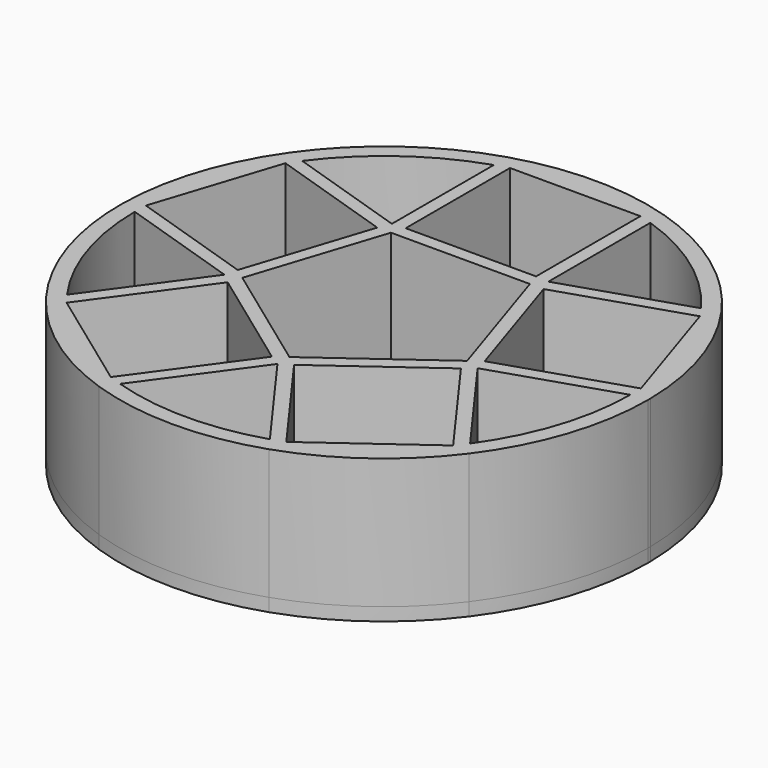
from build123d import *
from build123d import SkipClean  # not in build123d's __all__

# Parameters (mm, degrees)
F0_W     = 10
F0_H     = 10
F1_DEPTH = 1
F2_DEPTH = 10


with BuildPart() as f1:
    # F0 (on Top) → F1 (new body)
    with BuildSketch(Plane.XY):
        with BuildLine():
            Line((6, 8.2582915228), (6, 18.0277563773))
            ThreePointArc((6, 18.0277563773), (5.5020799323, 18.1859043333), (5, 18.3303027798))
            Line((5, 18.3303027798), (5, 8.3303027798))
            Line((5, 8.3303027798), (-5, 8.3303027798))
            Line((-5, 8.3303027798), (-5, 18.3303027798))
            ThreePointArc((-5, 18.3303027798), (-5.5020799323, 18.1859043333), (-6, 18.0277563773))
            Line((-6, 18.0277563773), (-6, 8.2582915228))
            Line((-6, 8.2582915228), (-5.1174302589, 7.9715272307))
            Line((-5.1174302589, 7.9715272307), (-5.3257767127, 7.3303027798))
            Line((-5.3257767127, 7.3303027798), (5.3257767127, 7.3303027798))
            Line((5.3257767127, 7.3303027798), (5.1174302589, 7.9715272307))
            Line((5.1174302589, 7.9715272307), (6, 8.2582915228))
        make_face()
        with BuildLine():
            ThreePointArc((-6.5079649301, -19.165254969), (0, -20.2400742479), (6.5079649301, -19.165254969))
            Line((6.5079649301, -19.165254969), (5.7423473643, -18.1114727935))
            ThreePointArc((5.7423473643, -18.1114727935), (0, -19), (-5.7423473643, -18.1114727935))
            Line((-5.7423473643, -18.1114727935), (-6.5079649301, -19.165254969))
        make_face()
        with BuildLine():
            ThreePointArc((-6.7291966722, -17.7684527224), (-6.2381301971, -17.9467471048), (-5.7423473643, -18.1114727935))
            Line((-5.7423473643, -18.1114727935), (0, -10.2078097002))
            Line((0, -10.2078097002), (-0.5454580974, -9.4570510365))
            Line((-0.5454580974, -9.4570510365), (0, -9.0607525315))
            Line((0, -9.0607525315), (-8.6172877376, -2.7999265141))
            Line((-8.6172877376, -2.7999265141), (-8.8256341914, -3.4411509649))
            Line((-8.8256341914, -3.4411509649), (-9.7082039325, -3.1543866727))
            Line((-9.7082039325, -3.1543866727), (-15.4505512968, -11.0580497659))
            ThreePointArc((-15.4505512968, -11.0580497659), (-15.1406825363, -11.4786642225), (-14.8193666159, -11.8906001995))
            Line((-14.8193666159, -11.8906001995), (-8.941514093, -3.8004302557))
            Line((-8.941514093, -3.8004302557), (-0.8513441492, -9.6782827786))
            Line((-0.8513441492, -9.6782827786), (-6.7291966722, -17.7684527224))
        make_face()
        Polygon((18.9782388763, 0.9090924895), (15.8880689325, 10.4196576525), (6.3775037696, 7.3294877087), (9.4676737133, -2.1810774542), align=None)
        Polygon((0, -9.0607525315), (8.6172877376, -2.7999265141), (5.3257767127, 7.3303027798), (-5.3257767127, 7.3303027798), (-8.6172877376, -2.7999265141), align=None)
        with BuildLine():
            Line((6, 8.2582915228), (15.2913132106, 11.2772221888))
            ThreePointArc((15.2913132106, 11.2772221888), (11.1679197936, 15.3713228931), (6, 18.0277563773))
            Line((6, 18.0277563773), (6, 8.2582915228))
        make_face()
        Polygon((-6.3775037696, 7.3294877087), (-15.8880689325, 10.4196576525), (-18.9782388763, 0.9090924895), (-9.4676737133, -2.1810774542), align=None)
        with BuildLine():
            ThreePointArc((16.2161688626, -12.1118319415), (19.2077727412, -6.3813847935), (20.2400742479, 0))
            ThreePointArc((20.2400742479, 0), (20.2396337779, 0.1335293897), (20.238312387, 0.2670529676))
            Line((20.238312387, 0.2670529676), (18.9995171431, -0.1354560067))
            ThreePointArc((18.9995171431, -0.1354560067), (18.0700738096, -5.8713228931), (15.4505512968, -11.0580497659))
            Line((15.4505512968, -11.0580497659), (16.2161688626, -12.1118319415))
        make_face()
        with BuildLine():
            ThreePointArc((14.8193666159, -11.8906001995), (15.1406825363, -11.4786642225), (15.4505512968, -11.0580497659))
            Line((15.4505512968, -11.0580497659), (9.7082039325, -3.1543866727))
            Line((9.7082039325, -3.1543866727), (8.8256341914, -3.4411509649))
            Line((8.8256341914, -3.4411509649), (8.6172877376, -2.7999265141))
            Line((8.6172877376, -2.7999265141), (0, -9.0607525315))
            Line((0, -9.0607525315), (0.5454580974, -9.4570510365))
            Line((0.5454580974, -9.4570510365), (0, -10.2078097002))
            Line((0, -10.2078097002), (5.7423473643, -18.1114727935))
            ThreePointArc((5.7423473643, -18.1114727935), (6.2381301971, -17.9467471048), (6.7291966722, -17.7684527224))
            Line((6.7291966722, -17.7684527224), (0.8513441492, -9.6782827786))
            Line((0.8513441492, -9.6782827786), (8.941514093, -3.8004302557))
            Line((8.941514093, -3.8004302557), (14.8193666159, -11.8906001995))
        make_face()
        with BuildLine():
            Line((-6, 18.0277563773), (-6, 19.3303027798))
            ThreePointArc((-6, 19.3303027798), (-11.8968171482, 16.3745640339), (-16.5301084545, 11.6797311631))
            Line((-16.5301084545, 11.6797311631), (-15.2913132106, 11.2772221888))
            ThreePointArc((-15.2913132106, 11.2772221888), (-11.1679197936, 15.3713228931), (-6, 18.0277563773))
        make_face()
        with BuildLine():
            ThreePointArc((-18.9995171431, -0.1354560067), (-18.0700738096, -5.8713228931), (-15.4505512968, -11.0580497659))
            Line((-15.4505512968, -11.0580497659), (-9.7082039325, -3.1543866727))
            Line((-9.7082039325, -3.1543866727), (-18.9995171431, -0.1354560067))
        make_face()
        with Locations((0, 13.3303027798)):
            Rectangle(F0_W, F0_H)
        with BuildLine():
            ThreePointArc((6.5079649301, -19.165254969), (11.8968171482, -16.3745640339), (16.2161688626, -12.1118319415))
            Line((16.2161688626, -12.1118319415), (6.5079649301, -19.165254969))
        make_face()
        with BuildLine():
            ThreePointArc((-16.2161688626, -12.1118319415), (-11.8968171482, -16.3745640339), (-6.5079649301, -19.165254969))
            Line((-6.5079649301, -19.165254969), (-16.2161688626, -12.1118319415))
        make_face()
        with BuildLine():
            Line((-20.238312387, 0.2670529676), (-16.5301084545, 11.6797311631))
            ThreePointArc((-16.5301084545, 11.6797311631), (-19.2494545037, 6.25452691), (-20.238312387, 0.2670529676))
        make_face()
        with BuildLine():
            Line((-6, 19.3303027798), (6, 19.3303027798))
            ThreePointArc((6, 19.3303027798), (0, 20.2400742479), (-6, 19.3303027798))
        make_face()
        with BuildLine():
            Line((16.5301084545, 11.6797311631), (20.238312387, 0.2670529676))
            ThreePointArc((20.238312387, 0.2670529676), (19.2494545037, 6.25452691), (16.5301084545, 11.6797311631))
        make_face()
        with BuildLine():
            Line((-15.2913132106, 11.2772221888), (-16.5301084545, 11.6797311631))
            Line((-16.5301084545, 11.6797311631), (-20.238312387, 0.2670529676))
            Line((-20.238312387, 0.2670529676), (-18.9995171431, -0.1354560067))
            ThreePointArc((-18.9995171431, -0.1354560067), (-18.9960590244, 0.3869645243), (-18.9782388763, 0.9090924895))
            ThreePointArc((-18.9782388763, 0.9090924895), (-18.0700738096, 5.8713228931), (-15.8880689325, 10.4196576525))
            ThreePointArc((-15.8880689325, 10.4196576525), (-15.5955866174, 10.8525424698), (-15.2913132106, 11.2772221888))
        make_face()
        Polygon((-14.8193666159, -11.8906001995), (-6.7291966722, -17.7684527224), (-0.8513441492, -9.6782827786), (-8.941514093, -3.8004302557), align=None)
        with BuildLine():
            Line((9.7082039325, -3.1543866727), (18.9995171431, -0.1354560067))
            ThreePointArc((18.9995171431, -0.1354560067), (18.9998792854, -0.0677284337), (19, 0))
            ThreePointArc((19, 0), (18.99455894, 0.4546764512), (18.9782388763, 0.9090924895))
            Line((18.9782388763, 0.9090924895), (9.4676737133, -2.1810774542))
            Line((9.4676737133, -2.1810774542), (6.3775037696, 7.3294877087))
            Line((6.3775037696, 7.3294877087), (15.8880689325, 10.4196576525))
            ThreePointArc((15.8880689325, 10.4196576525), (15.5955866174, 10.8525424698), (15.2913132106, 11.2772221888))
            Line((15.2913132106, 11.2772221888), (6, 8.2582915228))
            Line((6, 8.2582915228), (6, 7.3303027798))
            Line((6, 7.3303027798), (5.3257767127, 7.3303027798))
            Line((5.3257767127, 7.3303027798), (8.6172877376, -2.7999265141))
            Line((8.6172877376, -2.7999265141), (9.1627458351, -2.403628009))
            Line((9.1627458351, -2.403628009), (9.7082039325, -3.1543866727))
        make_face()
        with BuildLine():
            ThreePointArc((15.4505512968, -11.0580497659), (18.0700738096, -5.8713228931), (18.9995171431, -0.1354560067))
            Line((18.9995171431, -0.1354560067), (9.7082039325, -3.1543866727))
            Line((9.7082039325, -3.1543866727), (15.4505512968, -11.0580497659))
        make_face()
        with BuildLine():
            ThreePointArc((-20.238312387, 0.2670529676), (-19.2494545037, -6.25452691), (-16.2161688626, -12.1118319415))
            Line((-16.2161688626, -12.1118319415), (-15.4505512968, -11.0580497659))
            ThreePointArc((-15.4505512968, -11.0580497659), (-18.0700738096, -5.8713228931), (-18.9995171431, -0.1354560067))
            Line((-18.9995171431, -0.1354560067), (-20.238312387, 0.2670529676))
        make_face()
        with BuildLine():
            Line((-6, 8.2582915228), (-15.2913132106, 11.2772221888))
            ThreePointArc((-15.2913132106, 11.2772221888), (-15.5955866174, 10.8525424698), (-15.8880689325, 10.4196576525))
            Line((-15.8880689325, 10.4196576525), (-6.3775037696, 7.3294877087))
            Line((-6.3775037696, 7.3294877087), (-9.4676737133, -2.1810774542))
            Line((-9.4676737133, -2.1810774542), (-18.9782388763, 0.9090924895))
            ThreePointArc((-18.9782388763, 0.9090924895), (-18.9960590244, 0.3869645243), (-18.9995171431, -0.1354560067))
            Line((-18.9995171431, -0.1354560067), (-9.7082039325, -3.1543866727))
            Line((-9.7082039325, -3.1543866727), (-9.1627458351, -2.403628009))
            Line((-9.1627458351, -2.403628009), (-8.6172877376, -2.7999265141))
            Line((-8.6172877376, -2.7999265141), (-5.3257767127, 7.3303027798))
            Line((-5.3257767127, 7.3303027798), (-6, 7.3303027798))
            Line((-6, 7.3303027798), (-6, 8.2582915228))
        make_face()
        with BuildLine():
            Line((15.2913132106, 11.2772221888), (16.5301084545, 11.6797311631))
            ThreePointArc((16.5301084545, 11.6797311631), (11.8968171482, 16.3745640339), (6, 19.3303027798))
            Line((6, 19.3303027798), (6, 18.0277563773))
            ThreePointArc((6, 18.0277563773), (11.1679197936, 15.3713228931), (15.2913132106, 11.2772221888))
        make_face()
        Polygon((6.7291966722, -17.7684527224), (14.8193666159, -11.8906001995), (8.941514093, -3.8004302557), (0.8513441492, -9.6782827786), align=None)
        with BuildLine():
            ThreePointArc((-5.7423473643, -18.1114727935), (0, -19), (5.7423473643, -18.1114727935))
            Line((5.7423473643, -18.1114727935), (0, -10.2078097002))
            Line((0, -10.2078097002), (-5.7423473643, -18.1114727935))
        make_face()
        with BuildLine():
            Line((-6, 8.2582915228), (-6, 18.0277563773))
            ThreePointArc((-6, 18.0277563773), (-11.1679197936, 15.3713228931), (-15.2913132106, 11.2772221888))
            Line((-15.2913132106, 11.2772221888), (-6, 8.2582915228))
        make_face()
        with BuildLine():
            Line((18.9995171431, -0.1354560067), (20.238312387, 0.2670529676))
            Line((20.238312387, 0.2670529676), (16.5301084545, 11.6797311631))
            Line((16.5301084545, 11.6797311631), (15.2913132106, 11.2772221888))
            ThreePointArc((15.2913132106, 11.2772221888), (15.5955866174, 10.8525424698), (15.8880689325, 10.4196576525))
            ThreePointArc((15.8880689325, 10.4196576525), (18.0700738096, 5.8713228931), (18.9782388763, 0.9090924895))
            ThreePointArc((18.9782388763, 0.9090924895), (18.99455894, 0.4546764512), (19, 0))
            ThreePointArc((19, 0), (18.9998792854, -0.0677284337), (18.9995171431, -0.1354560067))
        make_face()
        with BuildLine():
            Line((6, 18.0277563773), (6, 19.3303027798))
            Line((6, 19.3303027798), (-6, 19.3303027798))
            Line((-6, 19.3303027798), (-6, 18.0277563773))
            ThreePointArc((-6, 18.0277563773), (-5.5020799323, 18.1859043333), (-5, 18.3303027798))
            ThreePointArc((-5, 18.3303027798), (0, 19), (5, 18.3303027798))
            ThreePointArc((5, 18.3303027798), (5.5020799323, 18.1859043333), (6, 18.0277563773))
        make_face()
        with BuildLine():
            Line((6.5079649301, -19.165254969), (16.2161688626, -12.1118319415))
            Line((16.2161688626, -12.1118319415), (15.4505512968, -11.0580497659))
            ThreePointArc((15.4505512968, -11.0580497659), (15.1406825363, -11.4786642225), (14.8193666159, -11.8906001995))
            ThreePointArc((14.8193666159, -11.8906001995), (11.1679197936, -15.3713228931), (6.7291966722, -17.7684527224))
            ThreePointArc((6.7291966722, -17.7684527224), (6.2381301971, -17.9467471048), (5.7423473643, -18.1114727935))
            Line((5.7423473643, -18.1114727935), (6.5079649301, -19.165254969))
        make_face()
        with BuildLine():
            Line((-16.2161688626, -12.1118319415), (-6.5079649301, -19.165254969))
            Line((-6.5079649301, -19.165254969), (-5.7423473643, -18.1114727935))
            ThreePointArc((-5.7423473643, -18.1114727935), (-6.2381301971, -17.9467471048), (-6.7291966722, -17.7684527224))
            ThreePointArc((-6.7291966722, -17.7684527224), (-11.1679197936, -15.3713228931), (-14.8193666159, -11.8906001995))
            ThreePointArc((-14.8193666159, -11.8906001995), (-15.1406825363, -11.4786642225), (-15.4505512968, -11.0580497659))
            Line((-15.4505512968, -11.0580497659), (-16.2161688626, -12.1118319415))
        make_face()
        with BuildLine():
            ThreePointArc((6.7291966722, -17.7684527224), (11.1679197936, -15.3713228931), (14.8193666159, -11.8906001995))
            Line((14.8193666159, -11.8906001995), (6.7291966722, -17.7684527224))
        make_face()
        with BuildLine():
            ThreePointArc((-14.8193666159, -11.8906001995), (-11.1679197936, -15.3713228931), (-6.7291966722, -17.7684527224))
            Line((-6.7291966722, -17.7684527224), (-14.8193666159, -11.8906001995))
        make_face()
        with BuildLine():
            Line((-18.9782388763, 0.9090924895), (-15.8880689325, 10.4196576525))
            ThreePointArc((-15.8880689325, 10.4196576525), (-18.0700738096, 5.8713228931), (-18.9782388763, 0.9090924895))
        make_face()
        with BuildLine():
            Line((-5, 18.3303027798), (5, 18.3303027798))
            ThreePointArc((5, 18.3303027798), (0, 19), (-5, 18.3303027798))
        make_face()
        with BuildLine():
            ThreePointArc((18.9782388763, 0.9090924895), (18.0700738096, 5.8713228931), (15.8880689325, 10.4196576525))
            Line((15.8880689325, 10.4196576525), (18.9782388763, 0.9090924895))
        make_face()
        Polygon((8.8256341914, -3.4411509649), (9.7082039325, -3.1543866727), (9.1627458351, -2.403628009), (8.6172877376, -2.7999265141), align=None)
        Polygon((6, 7.3303027798), (6, 8.2582915228), (5.1174302589, 7.9715272307), (5.3257767127, 7.3303027798), align=None)
        Polygon((-5.1174302589, 7.9715272307), (-6, 8.2582915228), (-6, 7.3303027798), (-5.3257767127, 7.3303027798), align=None)
        Polygon((-9.1627458351, -2.403628009), (-9.7082039325, -3.1543866727), (-8.8256341914, -3.4411509649), (-8.6172877376, -2.7999265141), align=None)
        Polygon((-0.5454580974, -9.4570510365), (0, -10.2078097002), (0.5454580974, -9.4570510365), (0, -9.0607525315), align=None)
    extrude(amount=-F1_DEPTH)

    # F0 (on Top) → F2 (join)
    with BuildSketch(Plane.XY):
        with BuildLine():
            Line((-6, 18.0277563773), (-6, 19.3303027798))
            ThreePointArc((-6, 19.3303027798), (-11.8968171482, 16.3745640339), (-16.5301084545, 11.6797311631))
            Line((-16.5301084545, 11.6797311631), (-15.2913132106, 11.2772221888))
            ThreePointArc((-15.2913132106, 11.2772221888), (-11.1679197936, 15.3713228931), (-6, 18.0277563773))
        make_face()
        with BuildLine():
            Line((6, 8.2582915228), (6, 18.0277563773))
            ThreePointArc((6, 18.0277563773), (5.5020799323, 18.1859043333), (5, 18.3303027798))
            Line((5, 18.3303027798), (5, 8.3303027798))
            Line((5, 8.3303027798), (-5, 8.3303027798))
            Line((-5, 8.3303027798), (-5, 18.3303027798))
            ThreePointArc((-5, 18.3303027798), (-5.5020799323, 18.1859043333), (-6, 18.0277563773))
            Line((-6, 18.0277563773), (-6, 8.2582915228))
            Line((-6, 8.2582915228), (-5.1174302589, 7.9715272307))
            Line((-5.1174302589, 7.9715272307), (-5.3257767127, 7.3303027798))
            Line((-5.3257767127, 7.3303027798), (5.3257767127, 7.3303027798))
            Line((5.3257767127, 7.3303027798), (5.1174302589, 7.9715272307))
            Line((5.1174302589, 7.9715272307), (6, 8.2582915228))
        make_face()
        with BuildLine():
            Line((-18.9782388763, 0.9090924895), (-15.8880689325, 10.4196576525))
            ThreePointArc((-15.8880689325, 10.4196576525), (-18.0700738096, 5.8713228931), (-18.9782388763, 0.9090924895))
        make_face()
        with BuildLine():
            Line((-5, 18.3303027798), (5, 18.3303027798))
            ThreePointArc((5, 18.3303027798), (0, 19), (-5, 18.3303027798))
        make_face()
        with BuildLine():
            ThreePointArc((18.9782388763, 0.9090924895), (18.0700738096, 5.8713228931), (15.8880689325, 10.4196576525))
            Line((15.8880689325, 10.4196576525), (18.9782388763, 0.9090924895))
        make_face()
        with BuildLine():
            Line((-20.238312387, 0.2670529676), (-16.5301084545, 11.6797311631))
            ThreePointArc((-16.5301084545, 11.6797311631), (-19.2494545037, 6.25452691), (-20.238312387, 0.2670529676))
        make_face()
        with BuildLine():
            Line((-6, 19.3303027798), (6, 19.3303027798))
            ThreePointArc((6, 19.3303027798), (0, 20.2400742479), (-6, 19.3303027798))
        make_face()
        with BuildLine():
            Line((16.5301084545, 11.6797311631), (20.238312387, 0.2670529676))
            ThreePointArc((20.238312387, 0.2670529676), (19.2494545037, 6.25452691), (16.5301084545, 11.6797311631))
        make_face()
        with BuildLine():
            Line((-15.2913132106, 11.2772221888), (-16.5301084545, 11.6797311631))
            Line((-16.5301084545, 11.6797311631), (-20.238312387, 0.2670529676))
            Line((-20.238312387, 0.2670529676), (-18.9995171431, -0.1354560067))
            ThreePointArc((-18.9995171431, -0.1354560067), (-18.9960590244, 0.3869645243), (-18.9782388763, 0.9090924895))
            ThreePointArc((-18.9782388763, 0.9090924895), (-18.0700738096, 5.8713228931), (-15.8880689325, 10.4196576525))
            ThreePointArc((-15.8880689325, 10.4196576525), (-15.5955866174, 10.8525424698), (-15.2913132106, 11.2772221888))
        make_face()
        with BuildLine():
            Line((9.7082039325, -3.1543866727), (18.9995171431, -0.1354560067))
            ThreePointArc((18.9995171431, -0.1354560067), (18.9998792854, -0.0677284337), (19, 0))
            ThreePointArc((19, 0), (18.99455894, 0.4546764512), (18.9782388763, 0.9090924895))
            Line((18.9782388763, 0.9090924895), (9.4676737133, -2.1810774542))
            Line((9.4676737133, -2.1810774542), (6.3775037696, 7.3294877087))
            Line((6.3775037696, 7.3294877087), (15.8880689325, 10.4196576525))
            ThreePointArc((15.8880689325, 10.4196576525), (15.5955866174, 10.8525424698), (15.2913132106, 11.2772221888))
            Line((15.2913132106, 11.2772221888), (6, 8.2582915228))
            Line((6, 8.2582915228), (6, 7.3303027798))
            Line((6, 7.3303027798), (5.3257767127, 7.3303027798))
            Line((5.3257767127, 7.3303027798), (8.6172877376, -2.7999265141))
            Line((8.6172877376, -2.7999265141), (9.1627458351, -2.403628009))
            Line((9.1627458351, -2.403628009), (9.7082039325, -3.1543866727))
        make_face()
        with BuildLine():
            Line((15.2913132106, 11.2772221888), (16.5301084545, 11.6797311631))
            ThreePointArc((16.5301084545, 11.6797311631), (11.8968171482, 16.3745640339), (6, 19.3303027798))
            Line((6, 19.3303027798), (6, 18.0277563773))
            ThreePointArc((6, 18.0277563773), (11.1679197936, 15.3713228931), (15.2913132106, 11.2772221888))
        make_face()
        with BuildLine():
            ThreePointArc((-20.238312387, 0.2670529676), (-19.2494545037, -6.25452691), (-16.2161688626, -12.1118319415))
            Line((-16.2161688626, -12.1118319415), (-15.4505512968, -11.0580497659))
            ThreePointArc((-15.4505512968, -11.0580497659), (-18.0700738096, -5.8713228931), (-18.9995171431, -0.1354560067))
            Line((-18.9995171431, -0.1354560067), (-20.238312387, 0.2670529676))
        make_face()
        with BuildLine():
            ThreePointArc((16.2161688626, -12.1118319415), (19.2077727412, -6.3813847935), (20.2400742479, 0))
            ThreePointArc((20.2400742479, 0), (20.2396337779, 0.1335293897), (20.238312387, 0.2670529676))
            Line((20.238312387, 0.2670529676), (18.9995171431, -0.1354560067))
            ThreePointArc((18.9995171431, -0.1354560067), (18.0700738096, -5.8713228931), (15.4505512968, -11.0580497659))
            Line((15.4505512968, -11.0580497659), (16.2161688626, -12.1118319415))
        make_face()
        with BuildLine():
            Line((-6, 8.2582915228), (-15.2913132106, 11.2772221888))
            ThreePointArc((-15.2913132106, 11.2772221888), (-15.5955866174, 10.8525424698), (-15.8880689325, 10.4196576525))
            Line((-15.8880689325, 10.4196576525), (-6.3775037696, 7.3294877087))
            Line((-6.3775037696, 7.3294877087), (-9.4676737133, -2.1810774542))
            Line((-9.4676737133, -2.1810774542), (-18.9782388763, 0.9090924895))
            ThreePointArc((-18.9782388763, 0.9090924895), (-18.9960590244, 0.3869645243), (-18.9995171431, -0.1354560067))
            Line((-18.9995171431, -0.1354560067), (-9.7082039325, -3.1543866727))
            Line((-9.7082039325, -3.1543866727), (-9.1627458351, -2.403628009))
            Line((-9.1627458351, -2.403628009), (-8.6172877376, -2.7999265141))
            Line((-8.6172877376, -2.7999265141), (-5.3257767127, 7.3303027798))
            Line((-5.3257767127, 7.3303027798), (-6, 7.3303027798))
            Line((-6, 7.3303027798), (-6, 8.2582915228))
        make_face()
        with BuildLine():
            Line((6, 18.0277563773), (6, 19.3303027798))
            Line((6, 19.3303027798), (-6, 19.3303027798))
            Line((-6, 19.3303027798), (-6, 18.0277563773))
            ThreePointArc((-6, 18.0277563773), (-5.5020799323, 18.1859043333), (-5, 18.3303027798))
            ThreePointArc((-5, 18.3303027798), (0, 19), (5, 18.3303027798))
            ThreePointArc((5, 18.3303027798), (5.5020799323, 18.1859043333), (6, 18.0277563773))
        make_face()
        with BuildLine():
            Line((18.9995171431, -0.1354560067), (20.238312387, 0.2670529676))
            Line((20.238312387, 0.2670529676), (16.5301084545, 11.6797311631))
            Line((16.5301084545, 11.6797311631), (15.2913132106, 11.2772221888))
            ThreePointArc((15.2913132106, 11.2772221888), (15.5955866174, 10.8525424698), (15.8880689325, 10.4196576525))
            ThreePointArc((15.8880689325, 10.4196576525), (18.0700738096, 5.8713228931), (18.9782388763, 0.9090924895))
            ThreePointArc((18.9782388763, 0.9090924895), (18.99455894, 0.4546764512), (19, 0))
            ThreePointArc((19, 0), (18.9998792854, -0.0677284337), (18.9995171431, -0.1354560067))
        make_face()
        Polygon((8.8256341914, -3.4411509649), (9.7082039325, -3.1543866727), (9.1627458351, -2.403628009), (8.6172877376, -2.7999265141), align=None)
        Polygon((6, 7.3303027798), (6, 8.2582915228), (5.1174302589, 7.9715272307), (5.3257767127, 7.3303027798), align=None)
        Polygon((-5.1174302589, 7.9715272307), (-6, 8.2582915228), (-6, 7.3303027798), (-5.3257767127, 7.3303027798), align=None)
        Polygon((-9.1627458351, -2.403628009), (-9.7082039325, -3.1543866727), (-8.8256341914, -3.4411509649), (-8.6172877376, -2.7999265141), align=None)
        Polygon((-0.5454580974, -9.4570510365), (0, -10.2078097002), (0.5454580974, -9.4570510365), (0, -9.0607525315), align=None)
        with BuildLine():
            Line((-16.2161688626, -12.1118319415), (-6.5079649301, -19.165254969))
            Line((-6.5079649301, -19.165254969), (-5.7423473643, -18.1114727935))
            ThreePointArc((-5.7423473643, -18.1114727935), (-6.2381301971, -17.9467471048), (-6.7291966722, -17.7684527224))
            ThreePointArc((-6.7291966722, -17.7684527224), (-11.1679197936, -15.3713228931), (-14.8193666159, -11.8906001995))
            ThreePointArc((-14.8193666159, -11.8906001995), (-15.1406825363, -11.4786642225), (-15.4505512968, -11.0580497659))
            Line((-15.4505512968, -11.0580497659), (-16.2161688626, -12.1118319415))
        make_face()
        with BuildLine():
            ThreePointArc((-6.7291966722, -17.7684527224), (-6.2381301971, -17.9467471048), (-5.7423473643, -18.1114727935))
            Line((-5.7423473643, -18.1114727935), (0, -10.2078097002))
            Line((0, -10.2078097002), (-0.5454580974, -9.4570510365))
            Line((-0.5454580974, -9.4570510365), (0, -9.0607525315))
            Line((0, -9.0607525315), (-8.6172877376, -2.7999265141))
            Line((-8.6172877376, -2.7999265141), (-8.8256341914, -3.4411509649))
            Line((-8.8256341914, -3.4411509649), (-9.7082039325, -3.1543866727))
            Line((-9.7082039325, -3.1543866727), (-15.4505512968, -11.0580497659))
            ThreePointArc((-15.4505512968, -11.0580497659), (-15.1406825363, -11.4786642225), (-14.8193666159, -11.8906001995))
            Line((-14.8193666159, -11.8906001995), (-8.941514093, -3.8004302557))
            Line((-8.941514093, -3.8004302557), (-0.8513441492, -9.6782827786))
            Line((-0.8513441492, -9.6782827786), (-6.7291966722, -17.7684527224))
        make_face()
        with BuildLine():
            ThreePointArc((-6.5079649301, -19.165254969), (0, -20.2400742479), (6.5079649301, -19.165254969))
            Line((6.5079649301, -19.165254969), (5.7423473643, -18.1114727935))
            ThreePointArc((5.7423473643, -18.1114727935), (0, -19), (-5.7423473643, -18.1114727935))
            Line((-5.7423473643, -18.1114727935), (-6.5079649301, -19.165254969))
        make_face()
        with BuildLine():
            ThreePointArc((6.5079649301, -19.165254969), (11.8968171482, -16.3745640339), (16.2161688626, -12.1118319415))
            Line((16.2161688626, -12.1118319415), (6.5079649301, -19.165254969))
        make_face()
        with BuildLine():
            ThreePointArc((-16.2161688626, -12.1118319415), (-11.8968171482, -16.3745640339), (-6.5079649301, -19.165254969))
            Line((-6.5079649301, -19.165254969), (-16.2161688626, -12.1118319415))
        make_face()
        with BuildLine():
            ThreePointArc((14.8193666159, -11.8906001995), (15.1406825363, -11.4786642225), (15.4505512968, -11.0580497659))
            Line((15.4505512968, -11.0580497659), (9.7082039325, -3.1543866727))
            Line((9.7082039325, -3.1543866727), (8.8256341914, -3.4411509649))
            Line((8.8256341914, -3.4411509649), (8.6172877376, -2.7999265141))
            Line((8.6172877376, -2.7999265141), (0, -9.0607525315))
            Line((0, -9.0607525315), (0.5454580974, -9.4570510365))
            Line((0.5454580974, -9.4570510365), (0, -10.2078097002))
            Line((0, -10.2078097002), (5.7423473643, -18.1114727935))
            ThreePointArc((5.7423473643, -18.1114727935), (6.2381301971, -17.9467471048), (6.7291966722, -17.7684527224))
            Line((6.7291966722, -17.7684527224), (0.8513441492, -9.6782827786))
            Line((0.8513441492, -9.6782827786), (8.941514093, -3.8004302557))
            Line((8.941514093, -3.8004302557), (14.8193666159, -11.8906001995))
        make_face()
        with BuildLine():
            ThreePointArc((6.7291966722, -17.7684527224), (11.1679197936, -15.3713228931), (14.8193666159, -11.8906001995))
            Line((14.8193666159, -11.8906001995), (6.7291966722, -17.7684527224))
        make_face()
        with BuildLine():
            ThreePointArc((-14.8193666159, -11.8906001995), (-11.1679197936, -15.3713228931), (-6.7291966722, -17.7684527224))
            Line((-6.7291966722, -17.7684527224), (-14.8193666159, -11.8906001995))
        make_face()
        with BuildLine():
            Line((6.5079649301, -19.165254969), (16.2161688626, -12.1118319415))
            Line((16.2161688626, -12.1118319415), (15.4505512968, -11.0580497659))
            ThreePointArc((15.4505512968, -11.0580497659), (15.1406825363, -11.4786642225), (14.8193666159, -11.8906001995))
            ThreePointArc((14.8193666159, -11.8906001995), (11.1679197936, -15.3713228931), (6.7291966722, -17.7684527224))
            ThreePointArc((6.7291966722, -17.7684527224), (6.2381301971, -17.9467471048), (5.7423473643, -18.1114727935))
            Line((5.7423473643, -18.1114727935), (6.5079649301, -19.165254969))
        make_face()
    with SkipClean():  # cleaning this boolean's faces spoils the solid; the shape is the same uncleaned
        extrude(amount=F2_DEPTH)


solid = f1.part
